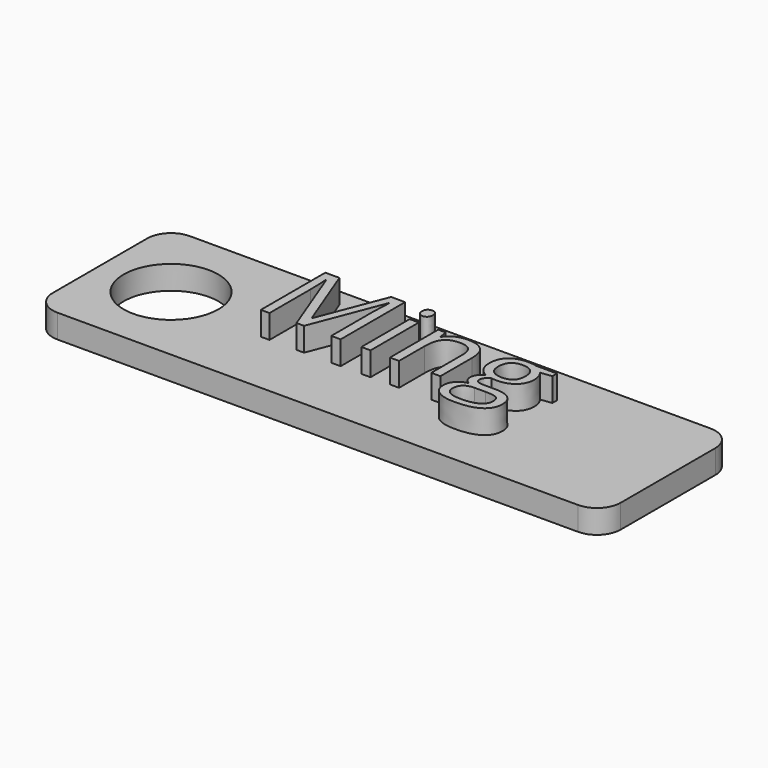
from build123d import *

# Parameters (mm, degrees)
F0_W         = 120
F0_H         = 35
F0_R         = 10
F1_DEPTH     = 5
F2_R         = 5
F3_TEXT_SIZE = 23.848685022
F4_DEPTH     = 5


# Not quite as in the source:
# - Text() gives the source's letters only with a copy of the font that has no kerning and outlines rounded to 1/6400 em; it was checked with that copy


with BuildPart() as f1:
    # F0 (on Top) → F1 (new body)
    with BuildSketch(Plane.XY):
        Rectangle(F0_W, F0_H)
        with Locations((-45, 0)):
            Circle(F0_R, mode=Mode.SUBTRACT)
    extrude(amount=F1_DEPTH)

    # F2
    f2_edges = [f1.edges().sort_by_distance(p)[0] for p in [
        (-60, 17.5, 2.5),
        (-60, -17.5, 2.5),
        (60, -17.5, 2.5),
        (60, 17.5, 2.5),
    ]]
    fillet(f2_edges, radius=F2_R)

    # F3 (on face) → F4 (join)
    with BuildSketch(Plane.XY.offset(5)):
        with Locations((-25.7565807551, -3.2565789297)):
            Text('Ming', F3_TEXT_SIZE, font='Open Sans', text_align=(TextAlign.LEFT, TextAlign.BOTTOM))
    extrude(amount=F4_DEPTH)


solid = f1.part
